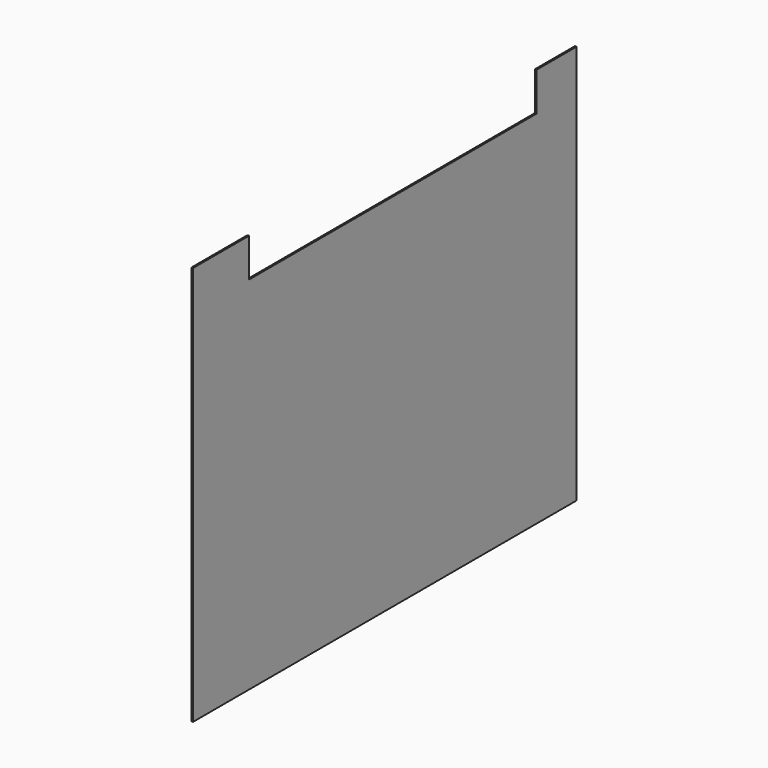
from build123d import *

# Parameters (mm, degrees)
F1_DEPTH = 1.5875


# Not quite as in the source:
# - a length typed as a fraction of an inch, garbled in the dataset ("3 / 203.2 mm" for 3/8 in), is restored


with BuildPart() as f1:
    # F0 (on Right) → F1 (new body)
    with BuildSketch(Plane.YZ):
        Polygon((-240, 200), (-240, -200), (240, -200), (240, 200), (190, 200), (190, 161.35), (-170, 161.35), (-170, 200), align=None)
    extrude(amount=F1_DEPTH)


solid = f1.part
